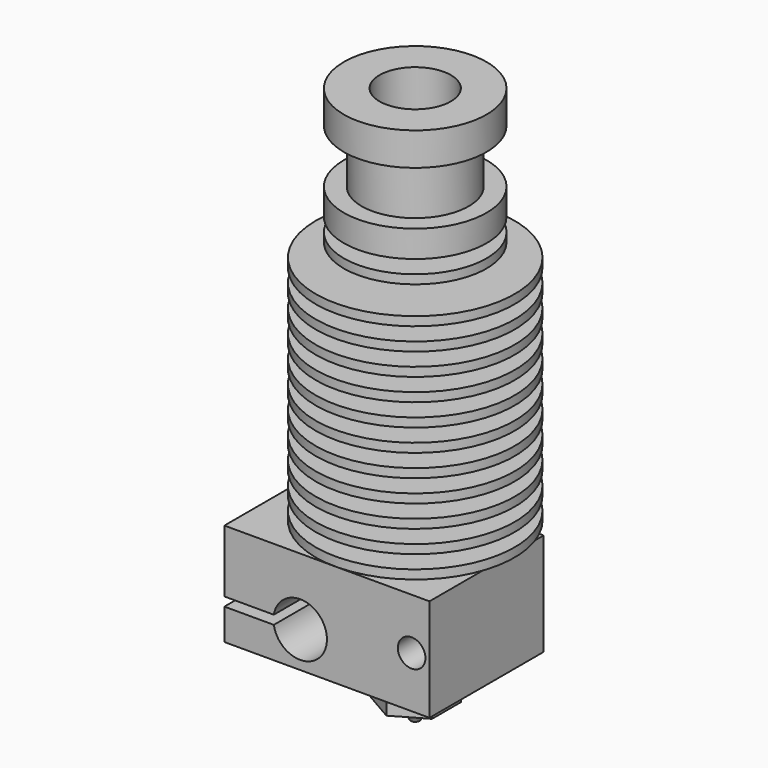
from build123d import *

# Parameters (mm, degrees)
F0_W      = 6
F0_H      = 6
F0_W_2    = 5
F0_H_2    = 1.5
F0_W_3    = 3
F0_H_3    = 1
F2_R      = 4
F3_DEPTH  = 6.5
F4_R      = 2.1
F5_DEPTH  = 50
F7_D      = 7
F7_DEPTH  = 15.1
F7_TIP    = 2.1030121666
F8_W      = 0.475
F8_H      = 2.1
F10_W     = 2
F10_H     = 4
F11_DEPTH = 8
F13_D     = 5
F13_DEPTH = 15.1
F13_TIP   = 1.5021515476
F15_D     = 2.5
F15_DEPTH = 21.5
F15_TIP   = 0.7510757738
F18_R     = 2.5
F18_R_2   = 2
F19_DEPTH = 3


with BuildPart() as f1:
    # F0 (on Front) → F1 (revolve)
    with BuildSketch(Plane.XZ):
        Polygon((-6, 0), (0, 0), (0, 3.7), (-8, 3.7), (-8, 0), align=None)
        with Locations((-3, -3)):
            Rectangle(F0_W, F0_H)
        Polygon((0, -14), (0, -13), (-5, -13), (-11.15, -13), (-11.15, -14), (-5, -14), align=None)
        with Locations((-2.5, -29.75)):
            Rectangle(F0_W_2, F0_H_2)
        with Locations((-2.5, -27.25)):
            Rectangle(F0_W_2, F0_H_2)
        Polygon((0, -39), (0, -38), (-5, -38), (-11.15, -38), (-11.15, -39), align=None)
        with Locations((-2.5, -9.75)):
            Rectangle(F0_W_2, F0_H_2)
        with Locations((-2.5, -32.25)):
            Rectangle(F0_W_2, F0_H_2)
        with Locations((-2.5, -19.75)):
            Rectangle(F0_W_2, F0_H_2)
        with Locations((-2.5, -22.25)):
            Rectangle(F0_W_2, F0_H_2)
        Polygon((0, -24), (0, -23), (-5, -23), (-11.15, -23), (-11.15, -24), (-5, -24), align=None)
        with Locations((-2.5, -17.25)):
            Rectangle(F0_W_2, F0_H_2)
        Polygon((0, -34), (0, -33), (-5, -33), (-11.15, -33), (-11.15, -34), (-5, -34), align=None)
        with Locations((-2.5, -24.75)):
            Rectangle(F0_W_2, F0_H_2)
        with Locations((-2.5, -34.75)):
            Rectangle(F0_W_2, F0_H_2)
        Polygon((0, -9), (0, -6), (-6, -6), (-8, -6), (-8, -9), (-5, -9), align=None)
        Polygon((0, -36.5), (0, -35.5), (-5, -35.5), (-11.15, -35.5), (-11.15, -36.5), (-5, -36.5), align=None)
        with Locations((-6.5, -11)):
            Rectangle(F0_W_3, F0_H_3)
        with Locations((-2.5, -14.75)):
            Rectangle(F0_W_2, F0_H_2)
        with Locations((-2.5, -12.25)):
            Rectangle(F0_W_2, F0_H_2)
        Polygon((0, -29), (0, -28), (-5, -28), (-11.15, -28), (-11.15, -29), (-5, -29), align=None)
        Polygon((0, -31.5), (0, -30.5), (-5, -30.5), (-11.15, -30.5), (-11.15, -31.5), (-5, -31.5), align=None)
        with Locations((-2.5, -11)):
            Rectangle(F0_W_2, F0_H_3)
        with Locations((-2.5, -37.25)):
            Rectangle(F0_W_2, F0_H_2)
        Polygon((0, -26.5), (0, -25.5), (-5, -25.5), (-11.15, -25.5), (-11.15, -26.5), (-5, -26.5), align=None)
        Polygon((0, -21.5), (0, -20.5), (-5, -20.5), (-11.15, -20.5), (-11.15, -21.5), (-5, -21.5), align=None)
        Polygon((0, -19), (0, -18), (-5, -18), (-11.15, -18), (-11.15, -19), (-5, -19), align=None)
        Polygon((0, -16.5), (0, -15.5), (-5, -15.5), (-11.15, -15.5), (-11.15, -16.5), (-5, -16.5), align=None)
    revolve(axis=Axis((0, 0, -3), (0, 0, -1)))

    # F2 (on face) → F3 (cut)
    with BuildSketch(Plane.XY.offset(3.7)):
        Circle(F2_R)
    extrude(amount=-F3_DEPTH, mode=Mode.SUBTRACT)

    # F4 (on face) → F5 (cut)
    with BuildSketch(Plane.XY.offset(-2.8)):
        Circle(F4_R)
    extrude(amount=-F5_DEPTH, mode=Mode.SUBTRACT)

    # F7
    with Locations(Plane(origin=(0, 0, -39), x_dir=(1, 0, 0), z_dir=(0, 0, -1))):
        with Locations((0, 0)):
            Hole(F7_D / 2, depth=F7_DEPTH)
            with Locations((0, 0, -(F7_DEPTH + F7_TIP / 2))):  # 118° drill point
                Cone(0, F7_D / 2, F7_TIP, mode=Mode.SUBTRACT)


with BuildPart() as f9:
    # F8 (on Front) → F9 (revolve)
    with BuildSketch(Plane.XZ):
        Polygon((-2.1, -26.9), (-2.1, -23.9), (-3.5, -23.9), (-3.5, -39), (-1.475, -39), (-1, -39), (-1, -28), align=None)
        with Locations((-1.2375, -40.05)):
            Rectangle(F8_W, F8_H)
        Polygon((-1, -46.1), (-1, -41.1), (-1.475, -41.1), (-3, -41.1), (-3, -46.1), align=None)
    revolve(axis=Axis((0, 0, -31.5), (0, 0, 1)))


with BuildPart() as f11:
    # F10 (on Front) → F11 (new body, symmetric)
    with BuildSketch(Plane.XZ):
        with BuildLine():
            Line((8, -41.1), (0, -41.1))
            Line((0, -41.1), (-15, -41.1))
            Line((-15, -41.1), (-15, -48.1))
            Line((-15, -48.1), (-9.4580398915, -48.1))
            ThreePointArc((-9.4580398915, -48.1), (-6.2491212192, -45.6105084316), (-3.5, -48.6))
            Line((-3.5, -48.6), (6, -48.6))
            Line((6, -48.6), (6, -48.4))
            ThreePointArc((6, -48.4), (4.9039844892, -45.7539844892), (7.55, -46.85))
            Line((7.55, -46.85), (8, -46.85))
            Line((8, -46.85), (8, -41.1))
        make_face()
        with BuildLine():
            Line((6, -52.6), (6, -48.6))
            Line((6, -48.6), (-3.5, -48.6))
            ThreePointArc((-3.5, -48.6), (-4.3786796564, -50.7213203436), (-6.5, -51.6))
            Line((-6.5, -51.6), (-6.5, -52.6))
            Line((-6.5, -52.6), (6, -52.6))
        make_face()
        with BuildLine():
            Line((-9.4580398915, -49.1), (-15, -49.1))
            Line((-15, -49.1), (-15, -52.6))
            Line((-15, -52.6), (-6.5, -52.6))
            Line((-6.5, -52.6), (-6.5, -51.6))
            ThreePointArc((-6.5, -51.6), (-8.4364916731, -50.8912878475), (-9.4580398915, -49.1))
        make_face()
        with Locations((7, -50.6)):
            Rectangle(F10_W, F10_H)
        with BuildLine():
            Line((8, -48.6), (8, -46.85))
            Line((8, -46.85), (7.55, -46.85))
            ThreePointArc((7.55, -46.85), (7.0960155108, -47.9460155108), (6, -48.4))
            Line((6, -48.4), (6, -48.6))
            Line((6, -48.6), (8, -48.6))
        make_face()
    extrude(amount=F11_DEPTH, both=True)

    # F13
    with Locations(Plane.XY.offset(-41.1)):
        with Locations((0, 0)):
            Hole(F13_D / 2, depth=F13_DEPTH)
            with Locations((0, 0, -(F13_DEPTH + F13_TIP / 2))):  # 118° drill point
                Cone(0, F13_D / 2, F13_TIP, mode=Mode.SUBTRACT)

    # F15
    with Locations(Plane.XY.offset(-41.1)):
        with Locations((-12.5, 0)):
            Hole(F15_D / 2, depth=F15_DEPTH)
            with Locations((0, 0, -(F15_DEPTH + F15_TIP / 2))):  # 118° drill point
                Cone(0, F15_D / 2, F15_TIP, mode=Mode.SUBTRACT)


with BuildPart() as f17:
    # F16 (on Front) → F17 (revolve)
    with BuildSketch(Plane.XZ):
        Polygon((-1, -52.1), (-1, -46.1), (-3, -46.1), (-3, -52.1), (-2.5, -52.1), align=None)
        Polygon((-1, -53.6), (-1, -52.1), (-2.5, -52.1), (-2.5, -53.6), (-2, -53.6), align=None)
        Polygon((-1, -56.6), (-1, -53.6), (-2, -53.6), (-2, -56.6), (-1.6547005384, -56.6), align=None)
        Polygon((-1, -56.6143593539), (-1, -56.6), (-1.6547005384, -56.6), (-0.5, -58.6), (-0.2, -58.6), (-0.2, -58), align=None)
    revolve(axis=Axis((0, 0, -52.35), (0, 0, -1)))

    # F18 (on face) → F19 (join)
    with BuildSketch(Plane(origin=(0, 0, -53.6), x_dir=(1, 0, 0), z_dir=(0, 0, -1))):
        Polygon((3.5, -2.0207259422), (3.5, 2.0207259422), (0, 4.0414518843), (-3.5, 2.0207259422), (-3.5, -2.0207259422), (0, -4.0414518843), align=None)
        Circle(F18_R, mode=Mode.SUBTRACT)
        Circle(F18_R)
        Circle(F18_R_2, mode=Mode.SUBTRACT)
    extrude(amount=F19_DEPTH)


solid = Compound([f1.part, f9.part, f11.part, f17.part])
